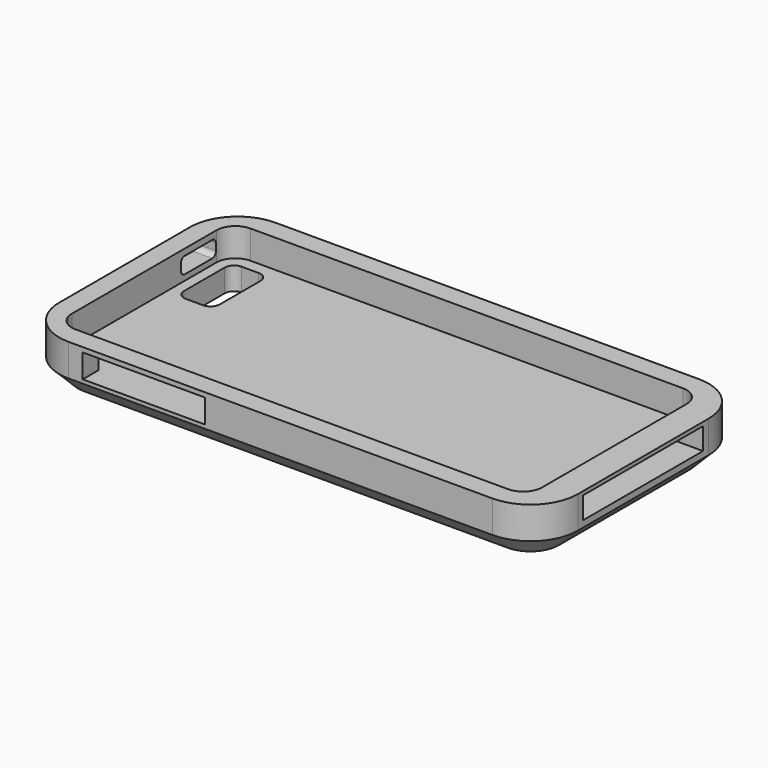
from build123d import *

# Parameters (mm, degrees)
F0_W      = 139.192
F0_H      = 69.342
F1_DEPTH  = 13.716
F2_W      = 123.698
F2_H      = 58.674
F3_DEPTH  = 7.62
F4_R      = 12.7
F5_R      = 12.7
F6_W      = 40.32391496
F6_H      = 5.8811781928
F7_DEPTH  = 25.4
F8_W      = 32.8259784728
F8_H      = 7.62
F9_DEPTH  = 25.4
F10_W     = 5.334
F10_H     = 1.2496084515
F11_DEPTH = 33.02
F12_W     = 9.6497610211
F12_H     = 18.7207064591
F13_DEPTH = 25.4
F14_R     = 2.54
F15_W     = 11.7547400296
F15_H     = 4.3837525882
F16_DEPTH = 25.4
F17_R     = 1.27
F18_SIZE  = 5.08
F19_DEPTH = 2.54
F20_R     = 5.08
F21_DEPTH = 1.778
F22_DEPTH = 1.778


with BuildPart() as f1:
    # F0 (on Top) → F1 (new body)
    with BuildSketch(Plane.XY):
        Rectangle(F0_W, F0_H)
    extrude(amount=F1_DEPTH)

    # F2 (on face) → F3 (cut)
    with BuildSketch(Plane.XY.offset(13.716)):
        Rectangle(F2_W, F2_H)
    extrude(amount=-F3_DEPTH, mode=Mode.SUBTRACT)

    # F4
    f4_edges = [f1.edges().sort_by_distance(p)[0] for p in [
        (69.596, -34.671, 6.858),
    ]]
    fillet(f4_edges, radius=F4_R)

    # F5
    f5_edges = [f1.edges().sort_by_distance(p)[0] for p in [
        (69.596, 34.671, 6.858),
        (-69.596, -34.671, 6.858),
        (-69.596, 34.671, 6.858),
    ]]
    fillet(f5_edges, radius=F5_R)

    # F6 (on face) → F7 (cut)
    with BuildSketch(Plane.YZ.offset(69.596)):
        with Locations((-0.1104911789, 9.7644287162)):
            Rectangle(F6_W, F6_H)
    extrude(amount=-F7_DEPTH, mode=Mode.SUBTRACT)

    # F8 (on face) → F9 (cut)
    with BuildSketch(Plane(origin=(0, -29.337, 0), x_dir=(-1, 0, 0), z_dir=(0, 1, 0))):
        with Locations((38.5076953098, 9.906)):
            Rectangle(F8_W, F8_H)
    extrude(amount=-F9_DEPTH, mode=Mode.SUBTRACT)

    # F10 (on face) → F11 (join)
    with BuildSketch(Plane.YZ.offset(-54.9206845462)):
        with Locations((-32.004, 13.0911957743)):
            Rectangle(F10_W, F10_H)
    extrude(amount=F11_DEPTH)

    # F12 (on face) → F13 (cut)
    with BuildSketch(Plane(origin=(0, 0, 0), x_dir=(1, 0, 0), z_dir=(0, 0, -1))):
        with Locations((-56.7813999951, -16.70263079)):
            Rectangle(F12_W, F12_H)
    extrude(amount=-F13_DEPTH, mode=Mode.SUBTRACT)

    # F14
    f14_edges = [f1.edges().sort_by_distance(p)[0] for p in [
        (-51.956519, 7.342278, 3.048),
        (-61.606281, 26.062984, 3.048),
        (-61.606281, 7.342278, 3.048),
        (-51.956519, 26.062984, 3.048),
    ]]
    fillet(f14_edges, radius=F14_R)

    # F15 (on face) → F16 (cut)
    with BuildSketch(Plane.YZ.offset(-61.849)):
        with Locations((18.2274878025, 9.8191385623)):
            Rectangle(F15_W, F15_H)
    extrude(amount=-F16_DEPTH, mode=Mode.SUBTRACT)

    # F17
    f17_edges = [f1.edges().sort_by_distance(p)[0] for p in [
        (-65.7225, 12.350118, 7.627262),
        (-65.7225, 12.350118, 12.011015),
        (-65.632225, 24.104858, 7.627262),
        (-65.632225, 24.104858, 12.011015),
    ]]
    fillet(f17_edges, radius=F17_R)

    # F18
    f18_edges = [f1.edges().sort_by_distance(p)[0] for p in [
        (0, -34.671, 0),
    ]]
    chamfer(f18_edges, length=F18_SIZE)

    # F19 (cut): a face of the model
    f19_faces = [f1.faces().sort_by_distance(p)[0] for p in [
        (-61.849, -2.3026136032, 9.916972896),
    ]]
    extrude(f19_faces, amount=-F19_DEPTH, mode=Mode.SUBTRACT)

    # F20
    f20_edges = [f1.edges().sort_by_distance(p)[0] for p in [
        (-64.389, -29.337, 9.906),
        (-64.389, 29.337, 9.906),
        (61.849, -29.337, 9.906),
        (61.849, 29.337, 9.906),
    ]]
    fillet(f20_edges, radius=F20_R)

    # F21 (add): a face of the model
    f21_faces = [f1.faces().sort_by_distance(p)[0] for p in [
        (-54.9206845462, -32.004, 9.2811957743),
    ]]
    extrude(f21_faces, amount=F21_DEPTH)

    # F22 (cut): a face of the model
    f22_faces = [f1.faces().sort_by_distance(p)[0] for p in [
        (-22.0947060734, -32.004, 9.2811957743),
    ]]
    extrude(f22_faces, amount=-F22_DEPTH, mode=Mode.SUBTRACT)


solid = f1.part
